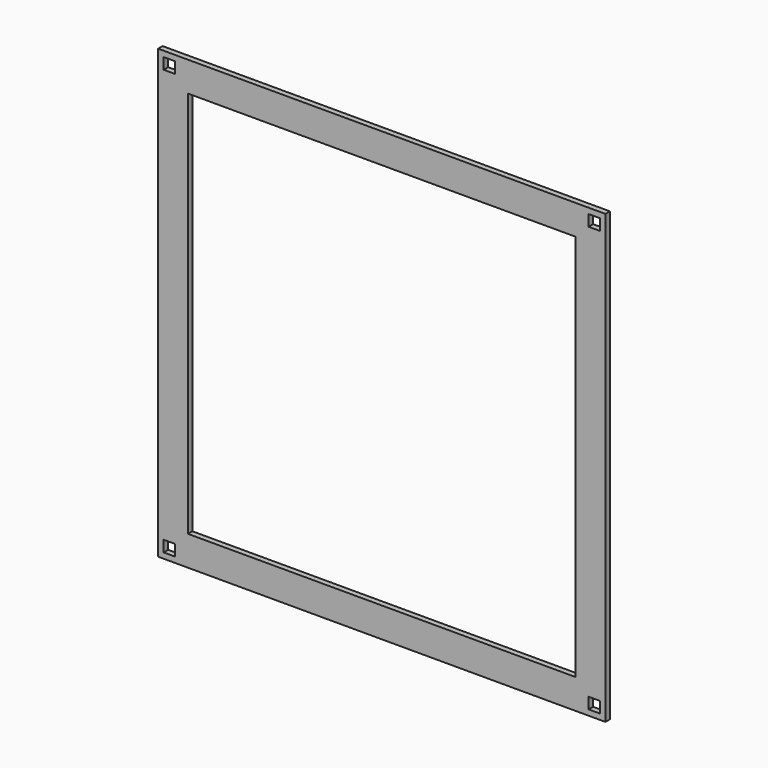
from build123d import *

# Parameters (mm, degrees)
F1_W     = 240
F1_H     = 240
F1_W_2   = 6
F1_H_2   = 6
F1_W_3   = 208
F1_H_3   = 208
F2_DEPTH = 3
F3_DEPTH = 25


with BuildPart() as f2:
    # F1 (on Front) → F2 (new body)
    with BuildSketch(Plane.XZ):
        with Locations((120, 120)):
            Rectangle(F1_W, F1_H)
        with Locations((6, 234)):
            Rectangle(F1_W_2, F1_H_2, mode=Mode.SUBTRACT)
        with Locations((120, 120)):
            Rectangle(F1_W_3, F1_H_3, mode=Mode.SUBTRACT)
        with Locations((6, 234)):
            Rectangle(F1_W_2, F1_H_2)
    extrude(amount=F2_DEPTH)

    # F1 (on Front) → F3 (cut)
    with BuildSketch(Plane.XZ):
        with Locations((6, 234)):
            Rectangle(F1_W_2, F1_H_2)
    extrude(amount=F3_DEPTH, mode=Mode.SUBTRACT)

    # F5: F2 across plane


with BuildPart() as f2_1:
    add(f2.part)
    add(f2.part.mirror(Plane(origin=(120, -1.5, 120), x_dir=(0, -1, 0), z_dir=(-1, 0, 0))), mode=Mode.INTERSECT)

    # F7: F2 across plane


with BuildPart() as f2_2:
    add(f2_1.part)
    add(f2_1.part.mirror(Plane(origin=(120, -1.5, 120), x_dir=(1, 0, 0), z_dir=(0, 0, 1))), mode=Mode.INTERSECT)


solid = f2_2.part
